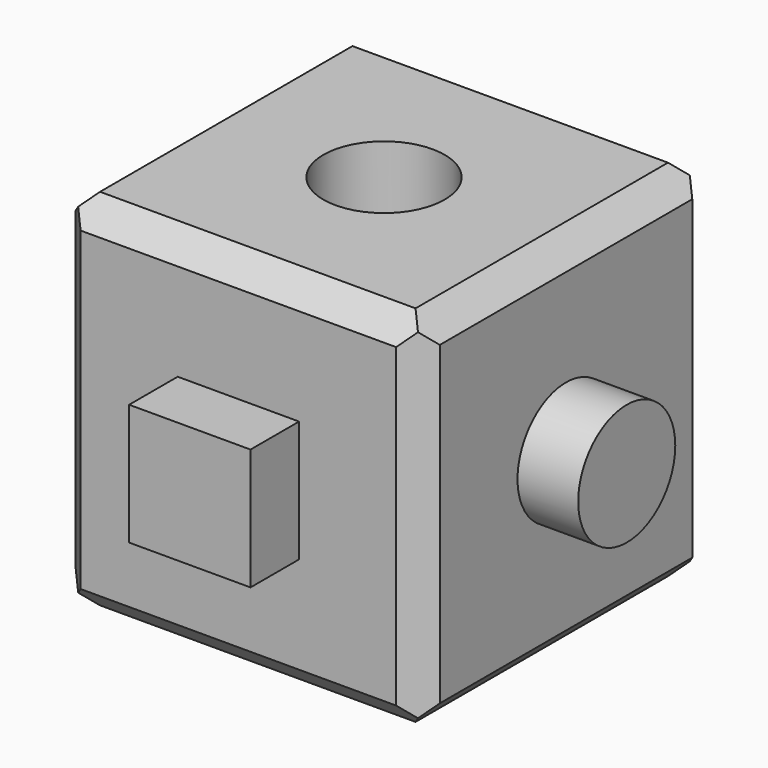
from build123d import *

# Parameters (mm, degrees)
F0_W     = 76.2
F0_H     = 76.2
F1_DEPTH = 76.2
F2_W     = 25.4
F2_H     = 25.4
F3_DEPTH = 12.7
F5_D     = 25.4
F6_R     = 12.7
F7_DEPTH = 12.7
F8_SIZE  = 5.08
F9_SIZE  = 5.08
F10_SIZE = 5.08
F11_SIZE = 5.08
F12_SIZE = 5.08
F13_SIZE = 5.08
F14_SIZE = 5.08
F15_SIZE = 5.08
F16_SIZE = 5.08
F17_SIZE = 5.08


# Not quite as in the source:
# - the program builds the solid bodies; features that only make, move or delete a surface that nothing else refers to are left out


with BuildPart() as f1:
    # F0 (on Front) → F1 (new body)
    with BuildSketch(Plane.XZ):
        with Locations((-38.1, 38.1)):
            Rectangle(F0_W, F0_H)
    extrude(amount=F1_DEPTH)

    # F2 (on face) → F3 (join)
    with BuildSketch(Plane.XZ.offset(76.2)):
        with Locations((-38.1, 38.1)):
            Rectangle(F2_W, F2_H)
    extrude(amount=F3_DEPTH)

    # F5 (through all)
    with Locations(Plane.XY.offset(76.2)):
        with Locations((-38.1, -38.1)):
            Hole(F5_D / 2)

    # F6 (on face) → F7 (join)
    with BuildSketch(Plane.YZ):
        with Locations((-38.1, 38.1)):
            Circle(F6_R)
    extrude(amount=F7_DEPTH)

    # F8
    f8_edges = [f1.edges().sort_by_distance(p)[0] for p in [
        (-38.1, -76.2, 76.2),
        (0, -38.1, 76.2),
    ]]
    chamfer(f8_edges, length=F8_SIZE)

    # F9
    f9_edges = [f1.edges().sort_by_distance(p)[0] for p in [
        (-40.64, 0, 76.2),
    ]]
    chamfer(f9_edges, length=F9_SIZE)

    # F10
    f10_edges = [f1.edges().sort_by_distance(p)[0] for p in [
        (-76.2, -38.1, 76.2),
    ]]
    chamfer(f10_edges, length=F10_SIZE)

    # F11
    f11_edges = [f1.edges().sort_by_distance(p)[0] for p in [
        (0, -76.2, 35.56),
        (-76.2, -76.2, 35.56),
    ]]
    chamfer(f11_edges, length=F11_SIZE)

    # F12
    f12_edges = [f1.edges().sort_by_distance(p)[0] for p in [
        (-38.1, -76.2, 0),
    ]]
    chamfer(f12_edges, length=F12_SIZE)

    # F13
    f13_edges = [f1.edges().sort_by_distance(p)[0] for p in [
        (0, -35.56, 0),
    ]]
    chamfer(f13_edges, length=F13_SIZE)

    # F14
    f14_edges = [f1.edges().sort_by_distance(p)[0] for p in [
        (0, 0, 38.1),
    ]]
    chamfer(f14_edges, length=F14_SIZE)

    # F15
    f15_edges = [f1.edges().sort_by_distance(p)[0] for p in [
        (-76.2, 0, 35.56),
    ]]
    chamfer(f15_edges, length=F15_SIZE)

    # F16
    f16_edges = [f1.edges().sort_by_distance(p)[0] for p in [
        (-76.2, -38.1, 0),
    ]]
    chamfer(f16_edges, length=F16_SIZE)

    # F17
    f17_edges = [f1.edges().sort_by_distance(p)[0] for p in [
        (-38.1, 0, 0),
    ]]
    chamfer(f17_edges, length=F17_SIZE)


solid = f1.part
